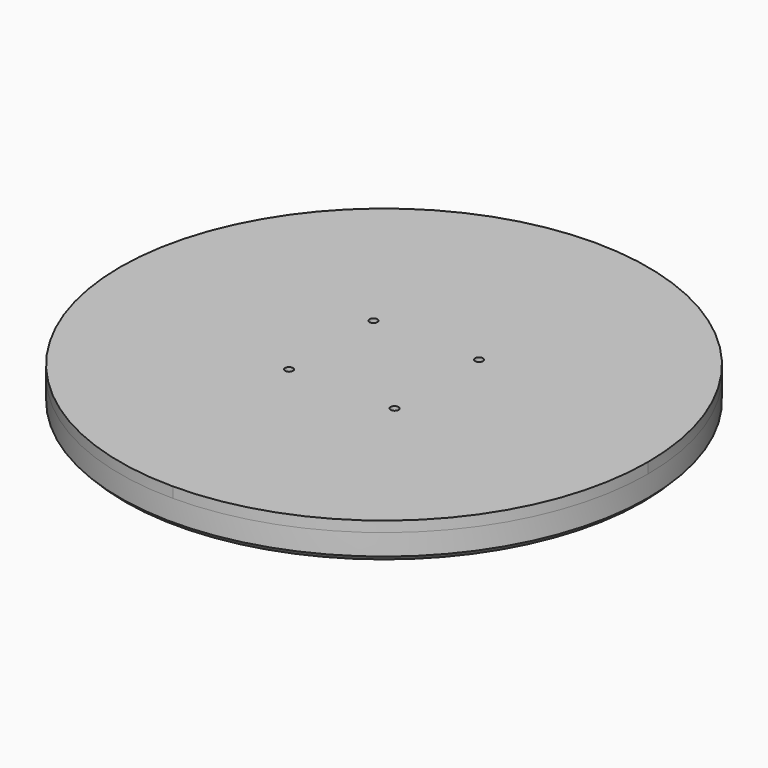
from build123d import *

# Parameters (mm, degrees)
F0_R            = 1.5
F1_DEPTH        = 4
F2_R            = 100
F2_R_2          = 90
F3_DEPTH        = 10
F4_SIZE         = 2
F6_DEPTH        = 10
F6_COPIES_COUNT = 65


# Not quite as in the source:
# - after a boolean that leaves OpenCascade's solid faulty, fix() repairs it
# - a feature of the source that left no trace in its solid (it failed there, or was rolled back) is left out
# - a pattern or mirror of a feature is missing from the dataset's text; its kind, count and spacing are read off the source's solid


with BuildPart() as f1:
    # F0 (on Top) → F1 (new body)
    with BuildSketch(Plane.XY):
        with BuildLine():
            Line((0, 0), (100, 0))
            ThreePointArc((100, 0), (70.7106781187, 70.7106781187), (0, 100))
            Line((0, 100), (0, 0))
        make_face()
        with Locations((20, 20)):
            Circle(F0_R, mode=Mode.SUBTRACT)
        with BuildLine():
            ThreePointArc((0, -100), (70.7106781187, -70.7106781187), (100, 0))
            Line((100, 0), (0, 0))
            Line((0, 0), (0, -100))
        make_face()
        with Locations((20, -20)):
            Circle(F0_R, mode=Mode.SUBTRACT)
        with BuildLine():
            Line((0, 0), (0, 100))
            ThreePointArc((0, 100), (-70.7106781187, 70.7106781187), (-100, 0))
            Line((-100, 0), (0, 0))
        make_face()
        with Locations((-20, 20)):
            Circle(F0_R, mode=Mode.SUBTRACT)
        with BuildLine():
            ThreePointArc((-100, 0), (-70.7106781187, -70.7106781187), (0, -100))
            Line((0, -100), (0, 0))
            Line((0, 0), (-100, 0))
        make_face()
        with Locations((-20, -20)):
            Circle(F0_R, mode=Mode.SUBTRACT)
    extrude(amount=F1_DEPTH)

    # F2 (on Top) → F3 (join)
    with BuildSketch(Plane.XY):
        Circle(F2_R)
        Circle(F2_R_2, mode=Mode.SUBTRACT)
    extrude(amount=-F3_DEPTH)

    # F4
    f4_edges = [f1.edges().sort_by_distance(p)[0] for p in [
        (-100, 0, -10),
    ]]
    chamfer(f4_edges, length=F4_SIZE)

    # F5 (on face) → F6 (cut)
    with BuildSketch(Plane(origin=(0, 0, -10), x_dir=(1, 0, 0), z_dir=(0, 0, -1))):
        with BuildLine():
            Line((3, 89.9499861034), (1.5304504731, 93.9875402452))
            ThreePointArc((1.5304504731, 93.9875402452), (0, 94.2795970069), (-1.5304504731, 93.9875402452))
            Line((-1.5304504731, 93.9875402452), (-3, 89.9499861034))
            ThreePointArc((-3, 89.9499861034), (0, 90), (3, 89.9499861034))
        make_face()
    f6 = extrude(amount=-F6_DEPTH, mode=Mode.SUBTRACT)

    add(f1.part.fix(), mode=Mode.REPLACE)

    # F6_copies: F6 ×65 about axis
    f6_copies_axis = Axis((0, 0, 0), (0, 0, 1))
    for i in range(1, F6_COPIES_COUNT):
        add(f6.rotate(f6_copies_axis, i * 360 / F6_COPIES_COUNT), mode=Mode.SUBTRACT)


solid = f1.part
